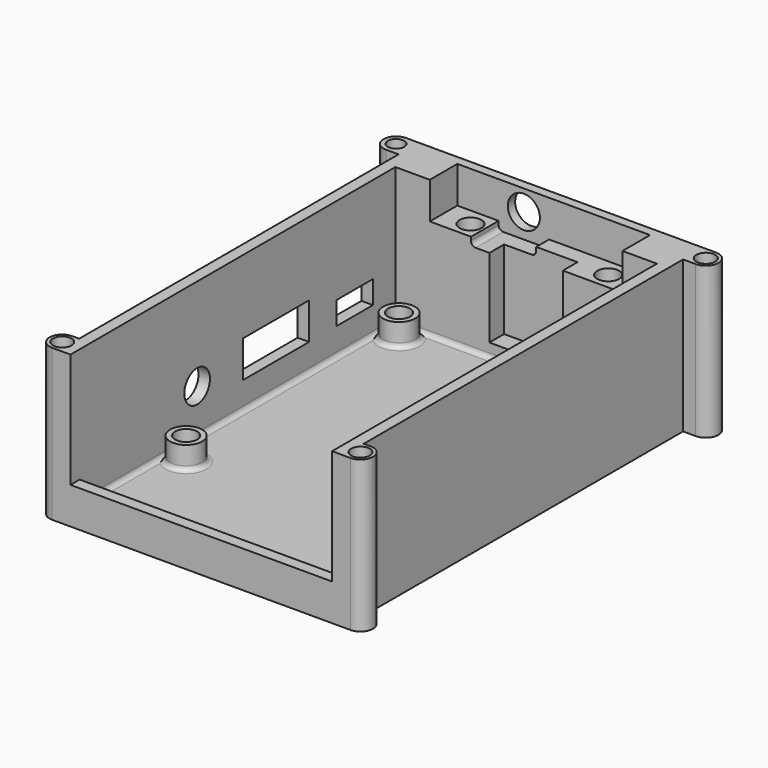
from build123d import *

# Parameters (mm, degrees)
F0_W         = 62
F0_H         = 91
F1_DEPTH     = 3
F2_W         = 62
F2_H         = 91
F2_W_2       = 57
F2_H_2       = 86
F3_DEPTH     = 30
F4_R         = 3.5
F5_DEPTH     = 5
F6_R         = 2.4
F7_DEPTH     = 3
F8_W         = 57
F8_H         = 25
F9_DEPTH     = 2.5
F10_W        = 18
F10_H        = 8
F10_R        = 3.5
F11_DEPTH    = 2.5
F12_DEPTH    = 7
F13_W        = 42
F13_H        = 7.5
F14_DEPTH    = 8
F15_R        = 2.4
F16_DEPTH    = 3
F17_W        = 11
F17_H        = 7.5
F18_DEPTH    = 1.8
F19_R        = 1
F20_R        = 3.5
F21_DEPTH    = 2
F22_T1_DEPTH = 62
F22_T3_DEPTH = 91
F24_DEPTH    = 33
F25_R        = 2.05
F25_R_2      = 1.7907732373
F26_DEPTH    = 4
F28_DEPTH    = 19


# Not quite as in the source:
# - a fillet or chamfer that OpenCascade refuses, or shapes differently, is made with other operations: its cross-section is extruded or revolved along the edge and cut away or added


with BuildPart() as f1:
    # F0 (on Top) → F1 (new body)
    with BuildSketch(Plane.XY):
        Rectangle(F0_W, F0_H)
    extrude(amount=F1_DEPTH)

    # F2 (on face) → F3 (join)
    with BuildSketch(Plane.XY.offset(3)):
        Rectangle(F2_W, F2_H)
        Rectangle(F2_W_2, F2_H_2, mode=Mode.SUBTRACT)
    extrude(amount=F3_DEPTH)

    # F4 (on face) → F5 (join)
    with BuildSketch(Plane.XY.offset(3)):
        with Locations((-24.5, 39)):
            Circle(F4_R)
        with Locations((24.5, 39)):
            Circle(F4_R)
        with Locations((-24.5, -19)):
            Circle(F4_R)
        with Locations((24.5, -19)):
            Circle(F4_R)
    extrude(amount=F5_DEPTH)

    # F6 (on face) → F7 (cut)
    with BuildSketch(Plane.XY.offset(8)):
        with Locations((-24.5, 39)):
            Circle(F6_R)
        with Locations((24.5, 39)):
            Circle(F6_R)
        with Locations((-24.5, -19)):
            Circle(F6_R)
        with Locations((24.5, -19)):
            Circle(F6_R)
    extrude(amount=-F7_DEPTH, mode=Mode.SUBTRACT)

    # F8 (on face) → F9 (cut, through all)
    with BuildSketch(Plane.XZ.offset(45.5)):
        with Locations((0, 20.5)):
            Rectangle(F8_W, F8_H)
    extrude(amount=-F9_DEPTH, mode=Mode.SUBTRACT)

    # F10 (on face) → F11 (cut, through all)
    with BuildSketch(Plane.YZ.offset(-28.5)):
        Polygon((26.9, 9), (36.9, 9), (36.9, 14), (31.9, 14), (26.9, 14), align=None)
        with Locations((10.5, 13)):
            Rectangle(F10_W, F10_H)
        with Locations((-11, 12.9)):
            Circle(F10_R)
    extrude(amount=-F11_DEPTH, mode=Mode.SUBTRACT)

    # F12 (add): a face of the model
    f12_faces = [f1.faces().sort_by_distance(p)[0] for p in [
        (0, 45.5, 16.5),
    ]]
    extrude(f12_faces, amount=F12_DEPTH)

    # F13 (on face) → F14 (cut)
    with BuildSketch(Plane.XY.offset(33)):
        with Locations((0, 46.75)):
            Rectangle(F13_W, F13_H)
    extrude(amount=-F14_DEPTH, mode=Mode.SUBTRACT)

    # F15 (on face) → F16 (cut)
    with BuildSketch(Plane.XY.offset(25)):
        with Locations((-15, 46.6)):
            Circle(F15_R)
        with Locations((15, 46.6)):
            Circle(F15_R)
    extrude(amount=-F16_DEPTH, mode=Mode.SUBTRACT)

    # F17 (on face) → F18 (cut)
    with BuildSketch(Plane.XY.offset(25)):
        with Locations((-6.5, 46.75)):
            Rectangle(F17_W, F17_H)
    extrude(amount=-F18_DEPTH, mode=Mode.SUBTRACT)

    # F19
    f19_edges = [f1.edges().sort_by_distance(p)[0] for p in [
        (-12, 46.75, 23.2),
        (-1, 46.75, 23.2),
    ]]
    fillet(f19_edges, radius=F19_R)

    # F20 (on face) → F21 (cut, through all)
    with BuildSketch(Plane.XZ.offset(-50.5)):
        with Locations((-6.5, 28.5)):
            Circle(F20_R)
    extrude(amount=-F21_DEPTH, mode=Mode.SUBTRACT)

    # F22: fillet of radius 1 on 8 edges, made by hand

    # F22_s2 → F22_t1 (join)
    with BuildSketch(Plane.YZ.offset(-31)):
        with BuildLine():
            ThreePointArc((43, 4), (42.7071067812, 3.2928932188), (42, 3))
            Line((42, 3), (43, 3))
            Line((43, 3), (43, 4))
        make_face()
        with BuildLine():
            ThreePointArc((-42, 3), (-42.7071067812, 3.2928932188), (-43, 4))
            Line((-43, 4), (-43, 3))
            Line((-43, 3), (-42, 3))
        make_face()
    extrude(amount=F22_T1_DEPTH)

    # F22_s4 → F22_t3 (join)
    with BuildSketch(Plane.XZ.offset(-45.5)):
        with BuildLine():
            ThreePointArc((-27.5, 3), (-28.2071067812, 3.2928932188), (-28.5, 4))
            Line((-28.5, 4), (-28.5, 3))
            Line((-28.5, 3), (-27.5, 3))
        make_face()
        with BuildLine():
            ThreePointArc((28.5, 4), (28.2071067812, 3.2928932188), (27.5, 3))
            Line((27.5, 3), (28.5, 3))
            Line((28.5, 3), (28.5, 4))
        make_face()
    extrude(amount=F22_T3_DEPTH)

    # F22_s5 → F22_t6 (revolve)
    with BuildSketch(Plane.XZ.offset(-39)):
        with BuildLine():
            ThreePointArc((29, 3), (28.2928932188, 3.2928932188), (28, 4))
            Line((28, 4), (28, 3))
            Line((28, 3), (29, 3))
        make_face()
    revolve(axis=Axis((24.5, 39, 3), (0, 0, 1)))

    # F22_s7 → F22_t8 (revolve)
    with BuildSketch(Plane.XZ.offset(-39)):
        with BuildLine():
            ThreePointArc((-20, 3), (-20.7071067812, 3.2928932188), (-21, 4))
            Line((-21, 4), (-21, 3))
            Line((-21, 3), (-20, 3))
        make_face()
    revolve(axis=Axis((-24.5, 39, 3), (0, 0, 1)))

    # F22_s9 → F22_t10 (revolve)
    with BuildSketch(Plane.XZ.offset(19)):
        with BuildLine():
            ThreePointArc((-20, 3), (-20.7071067812, 3.2928932188), (-21, 4))
            Line((-21, 4), (-21, 3))
            Line((-21, 3), (-20, 3))
        make_face()
    revolve(axis=Axis((-24.5, -19, 3), (0, 0, 1)))

    # F22_s11 → F22_t12 (revolve)
    with BuildSketch(Plane.XZ.offset(19)):
        with BuildLine():
            ThreePointArc((29, 3), (28.2928932188, 3.2928932188), (28, 4))
            Line((28, 4), (28, 3))
            Line((28, 3), (29, 3))
        make_face()
    revolve(axis=Axis((24.5, -19, 3), (0, 0, 1)))

    # F23 (on face) → F24 (join, through all)
    with BuildSketch(Plane.XY):
        with BuildLine():
            Line((31, -45.5), (32.5, -45.5))
            ThreePointArc((32.5, -45.5), (35.25, -42.75), (32.5, -40))
            Line((32.5, -40), (31, -40))
            Line((31, -40), (31, -45.5))
        make_face()
        with BuildLine():
            Line((-31, -40), (-32.5, -40))
            ThreePointArc((-32.5, -40), (-35.25, -42.75), (-32.5, -45.5))
            Line((-32.5, -45.5), (-31, -45.5))
            Line((-31, -45.5), (-31, -40))
        make_face()
        with BuildLine():
            Line((-31, 52.5), (-33.75, 52.5))
            ThreePointArc((-33.75, 52.5), (-36.5, 49.75), (-33.75, 47))
            Line((-33.75, 47), (-31, 47))
            Line((-31, 47), (-31, 52.5))
        make_face()
        with BuildLine():
            Line((31, 47), (33.75, 47))
            ThreePointArc((33.75, 47), (36.5, 49.75), (33.75, 52.5))
            Line((33.75, 52.5), (31, 52.5))
            Line((31, 52.5), (31, 47))
        make_face()
    extrude(amount=F24_DEPTH)

    # F25 (on face) → F26 (cut)
    with BuildSketch(Plane.XY.offset(33)):
        with Locations((-32.5, -42.75)):
            Circle(F25_R)
        with Locations((32.5, -42.75)):
            Circle(F25_R)
        with Locations((-33.75, 49.75)):
            Circle(F25_R_2)
        with Locations((33.75, 49.75)):
            Circle(F25_R)
    extrude(amount=-F26_DEPTH, mode=Mode.SUBTRACT)

    # F27 (on face) → F28 (cut, through all)
    with BuildSketch(Plane.XY.offset(25)):
        Polygon((-8, 43), (8, 43), (8, 47), (0, 47), (-8, 47), align=None)
    extrude(amount=-F28_DEPTH, mode=Mode.SUBTRACT)


solid = f1.part
